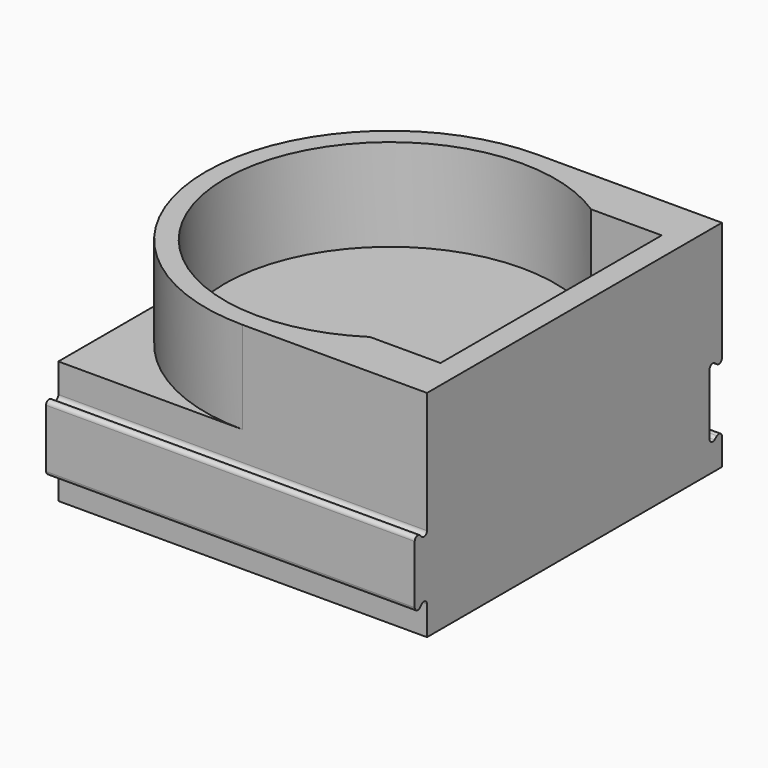
from build123d import *

# Parameters (mm, degrees)
F1_DEPTH  = 16
F2_DEPTH  = 12
F3_W      = 44
F3_H      = 44
F4_DEPTH  = 2
F5_R      = 1.65
F6_DEPTH  = 25
F8_DEPTH  = 48
F9_DEPTH  = 48
F10_R     = 0.5
F11_W     = 1.8
F11_H     = 2.1
F14_DEPTH = 10


# Not quite as in the source:
# - a feature names something its author has since deleted; it is built from what else it names


with BuildPart() as f1:
    # F0 (on Top) → F1 (new body)
    with BuildSketch(Plane.XY):
        with BuildLine():
            ThreePointArc((0, 24), (8.4852813742, 22.4499443206), (15.8745078664, 18))
            Line((15.8745078664, 18), (20.9579760163, 18))
            Line((20.9579760163, 18), (20.9579760163, 11.6945817069))
            ThreePointArc((20.9579760163, 11.6945817069), (23.2270469969, 6.0418778376), (24, 0))
            Line((24, 0), (24, 24))
            Line((24, 24), (0, 24))
        make_face()
        with BuildLine():
            Line((20.9579760163, -18), (15.8745078664, -18))
            ThreePointArc((15.8745078664, -18), (8.4852813742, -22.4499443206), (0, -24))
            Line((0, -24), (24, -24))
            Line((24, -24), (24, 0))
            ThreePointArc((24, 0), (23.2270469969, -6.0418778376), (20.9579760163, -11.6945817069))
            Line((20.9579760163, -11.6945817069), (20.9579760163, -18))
        make_face()
        with BuildLine():
            Line((15.8745078664, 18), (11.7579760163, 18))
            ThreePointArc((11.7579760163, 18), (17.6397784352, 12.2917946922), (20.9579760163, 4.7972118256))
            Line((20.9579760163, 4.7972118256), (20.9579760163, 11.6945817069))
            ThreePointArc((20.9579760163, 11.6945817069), (18.6841521671, 15.0632817737), (15.8745078664, 18))
        make_face()
        with BuildLine():
            ThreePointArc((11.7579760163, -18), (-21.5, 0), (11.7579760163, 18))
            Line((11.7579760163, 18), (15.8745078664, 18))
            ThreePointArc((15.8745078664, 18), (8.4852813742, 22.4499443206), (0, 24))
            ThreePointArc((0, 24), (-16.9705627485, 16.9705627485), (-24, 0))
            ThreePointArc((-24, 0), (-16.9705627485, -16.9705627485), (0, -24))
            ThreePointArc((0, -24), (8.4852813742, -22.4499443206), (15.8745078664, -18))
            Line((15.8745078664, -18), (11.7579760163, -18))
        make_face()
        with BuildLine():
            ThreePointArc((20.9579760163, -4.7972118256), (17.6397784352, -12.2917946922), (11.7579760163, -18))
            Line((11.7579760163, -18), (15.8745078664, -18))
            ThreePointArc((15.8745078664, -18), (18.6841521671, -15.0632817737), (20.9579760163, -11.6945817069))
            Line((20.9579760163, -11.6945817069), (20.9579760163, -4.7972118256))
        make_face()
        with BuildLine():
            Line((20.9579760163, 11.6945817069), (20.9579760163, 4.7972118256))
            ThreePointArc((20.9579760163, 4.7972118256), (21.364064271, 2.4138678143), (21.5, 0))
            ThreePointArc((21.5, 0), (21.364064271, -2.4138678143), (20.9579760163, -4.7972118256))
            Line((20.9579760163, -4.7972118256), (20.9579760163, -11.6945817069))
            ThreePointArc((20.9579760163, -11.6945817069), (23.2270469969, -6.0418778376), (24, 0))
            ThreePointArc((24, 0), (23.2270469969, 6.0418778376), (20.9579760163, 11.6945817069))
        make_face()
        with BuildLine():
            ThreePointArc((-24, 0), (-16.9705627485, 16.9705627485), (0, 24))
            Line((0, 24), (-24, 24))
            Line((-24, 24), (-24, 0))
        make_face()
        with BuildLine():
            Line((11.7579760163, -18), (11.7579760163, 18))
            ThreePointArc((11.7579760163, 18), (-21.5, 0), (11.7579760163, -18))
        make_face()
        with BuildLine():
            Line((-24, -24), (0, -24))
            ThreePointArc((0, -24), (-16.9705627485, -16.9705627485), (-24, 0))
            Line((-24, 0), (-24, -24))
        make_face()
        with BuildLine():
            Line((20.9579760163, 18), (15.8745078664, 18))
            ThreePointArc((15.8745078664, 18), (18.6841521671, 15.0632817737), (20.9579760163, 11.6945817069))
            Line((20.9579760163, 11.6945817069), (20.9579760163, 18))
        make_face()
        with BuildLine():
            ThreePointArc((20.9579760163, -11.6945817069), (18.6841521671, -15.0632817737), (15.8745078664, -18))
            Line((15.8745078664, -18), (20.9579760163, -18))
            Line((20.9579760163, -18), (20.9579760163, -11.6945817069))
        make_face()
        with BuildLine():
            ThreePointArc((21.5, 0), (21.364064271, 2.4138678143), (20.9579760163, 4.7972118256))
            Line((20.9579760163, 4.7972118256), (20.9579760163, -4.7972118256))
            ThreePointArc((20.9579760163, -4.7972118256), (21.364064271, -2.4138678143), (21.5, 0))
        make_face()
        with BuildLine():
            ThreePointArc((20.9579760163, 4.7972118256), (17.6397784352, 12.2917946922), (11.7579760163, 18))
            Line((11.7579760163, 18), (11.7579760163, -18))
            ThreePointArc((11.7579760163, -18), (17.6397784352, -12.2917946922), (20.9579760163, -4.7972118256))
            Line((20.9579760163, -4.7972118256), (20.9579760163, 4.7972118256))
        make_face()
    extrude(amount=-F1_DEPTH)

    # F0 (on Top) → F2 (join)
    with BuildSketch(Plane.XY):
        with BuildLine():
            ThreePointArc((11.7579760163, -18), (-21.5, 0), (11.7579760163, 18))
            Line((11.7579760163, 18), (15.8745078664, 18))
            ThreePointArc((15.8745078664, 18), (8.4852813742, 22.4499443206), (0, 24))
            ThreePointArc((0, 24), (-16.9705627485, 16.9705627485), (-24, 0))
            ThreePointArc((-24, 0), (-16.9705627485, -16.9705627485), (0, -24))
            ThreePointArc((0, -24), (8.4852813742, -22.4499443206), (15.8745078664, -18))
            Line((15.8745078664, -18), (11.7579760163, -18))
        make_face()
        with BuildLine():
            Line((20.9579760163, -18), (15.8745078664, -18))
            ThreePointArc((15.8745078664, -18), (8.4852813742, -22.4499443206), (0, -24))
            Line((0, -24), (24, -24))
            Line((24, -24), (24, 0))
            ThreePointArc((24, 0), (23.2270469969, -6.0418778376), (20.9579760163, -11.6945817069))
            Line((20.9579760163, -11.6945817069), (20.9579760163, -18))
        make_face()
        with BuildLine():
            Line((20.9579760163, 11.6945817069), (20.9579760163, 4.7972118256))
            ThreePointArc((20.9579760163, 4.7972118256), (21.364064271, 2.4138678143), (21.5, 0))
            ThreePointArc((21.5, 0), (21.364064271, -2.4138678143), (20.9579760163, -4.7972118256))
            Line((20.9579760163, -4.7972118256), (20.9579760163, -11.6945817069))
            ThreePointArc((20.9579760163, -11.6945817069), (23.2270469969, -6.0418778376), (24, 0))
            ThreePointArc((24, 0), (23.2270469969, 6.0418778376), (20.9579760163, 11.6945817069))
        make_face()
        with BuildLine():
            ThreePointArc((0, 24), (8.4852813742, 22.4499443206), (15.8745078664, 18))
            Line((15.8745078664, 18), (20.9579760163, 18))
            Line((20.9579760163, 18), (20.9579760163, 11.6945817069))
            ThreePointArc((20.9579760163, 11.6945817069), (23.2270469969, 6.0418778376), (24, 0))
            Line((24, 0), (24, 24))
            Line((24, 24), (0, 24))
        make_face()
        with BuildLine():
            ThreePointArc((21.5, 0), (21.364064271, 2.4138678143), (20.9579760163, 4.7972118256))
            Line((20.9579760163, 4.7972118256), (20.9579760163, -4.7972118256))
            ThreePointArc((20.9579760163, -4.7972118256), (21.364064271, -2.4138678143), (21.5, 0))
        make_face()
    extrude(amount=F2_DEPTH)

    # F3 (on face) → F4 (cut)
    with BuildSketch(Plane(origin=(0, 0, -16), x_dir=(1, 0, 0), z_dir=(0, 0, -1))):
        Rectangle(F3_W, F3_H)
    extrude(amount=-F4_DEPTH, mode=Mode.SUBTRACT)

    # F5 (on face) → F6 (cut)
    with BuildSketch(Plane(origin=(0, 0, -14), x_dir=(1, 0, 0), z_dir=(0, 0, -1))):
        with BuildLine():
            ThreePointArc((17.3732751343, 12.6656745224), (16.7780906851, 13.4441687345), (16.1480507184, 14.1947334599))
            ThreePointArc((16.1480507184, 14.1947334599), (14.4166793265, 11.5940731357), (17.3745826654, 12.6))
            ThreePointArc((17.3745826654, 12.6), (17.3742557502, 12.6328437686), (17.3732751343, 12.6656745224))
        make_face()
        with BuildLine():
            ThreePointArc((17.3732751343, 12.6656745224), (17.0122035784, 13.6317617866), (16.1480507184, 14.1947334599))
            ThreePointArc((16.1480507184, 14.1947334599), (16.7780906851, 13.4441687345), (17.3732751343, 12.6656745224))
        make_face()
        with Locations((15.7245826654, 6.3)):
            Circle(F5_R)
        with Locations((15.7245826654, 0)):
            Circle(F5_R)
        with Locations((15.7245826654, -6.3)):
            Circle(F5_R)
        with BuildLine():
            ThreePointArc((17.3732751343, -12.6656745224), (16.7780906851, -13.4441687345), (16.1480507184, -14.1947334599))
            ThreePointArc((16.1480507184, -14.1947334599), (17.0122035784, -13.6317617866), (17.3732751343, -12.6656745224))
        make_face()
        with BuildLine():
            ThreePointArc((17.3745826654, -12.6), (14.4166793265, -11.5940731357), (16.1480507184, -14.1947334599))
            ThreePointArc((16.1480507184, -14.1947334599), (16.7780906851, -13.4441687345), (17.3732751343, -12.6656745224))
            ThreePointArc((17.3732751343, -12.6656745224), (17.3742557502, -12.6328437686), (17.3745826654, -12.6))
        make_face()
    extrude(amount=-F6_DEPTH, mode=Mode.SUBTRACT)

    # F7 (on face) → F8 (join, through all)
    with BuildSketch(Plane.YZ.offset(24)):
        Polygon((-26, -13), (-24, -11), (-24, -5), (-26, -3), align=None)
    extrude(amount=-F8_DEPTH)

    # F7 (on face) → F9 (cut, through all)
    with BuildSketch(Plane.YZ.offset(24)):
        Polygon((22, -13), (24, -11.4928918998), (24, -4.5071081002), (22, -3), align=None)
    extrude(amount=-F9_DEPTH, mode=Mode.SUBTRACT)

    # F10
    f10_edges = [f1.edges().sort_by_distance(p)[0] for p in [
        (0, -26, -13),
        (0, -26, -3),
        (0, 22, -3),
        (0, 22, -13),
        (0, 24, -4.507108),
        (0, 24, -11.492892),
        (0, -24, -5),
        (0, -24, -11),
    ]]
    fillet(f10_edges, radius=F10_R)

    # F11 (on Front) → F12 (revolve, cut)
    with BuildSketch(Plane.XZ):
        with Locations((12.6579760163, 5.05)):
            Rectangle(F11_W, F11_H)
    revolve(axis=Axis((0, 0, 12), (0, 0, -1)), mode=Mode.SUBTRACT)

    # F0 (on Top) + F13 (on face) → F14 (cut)
    with BuildSketch(Plane.XY):
        with BuildLine():
            ThreePointArc((20.9579760163, 4.7972118256), (17.6397784352, 12.2917946922), (11.7579760163, 18))
            Line((11.7579760163, 18), (11.7579760163, -18))
            ThreePointArc((11.7579760163, -18), (17.6397784352, -12.2917946922), (20.9579760163, -4.7972118256))
            Line((20.9579760163, -4.7972118256), (20.9579760163, 4.7972118256))
        make_face()
        with BuildLine():
            ThreePointArc((20.9579760163, -4.7972118256), (17.6397784352, -12.2917946922), (11.7579760163, -18))
            Line((11.7579760163, -18), (15.8745078664, -18))
            ThreePointArc((15.8745078664, -18), (18.6841521671, -15.0632817737), (20.9579760163, -11.6945817069))
            Line((20.9579760163, -11.6945817069), (20.9579760163, -4.7972118256))
        make_face()
        with BuildLine():
            ThreePointArc((20.9579760163, -11.6945817069), (18.6841521671, -15.0632817737), (15.8745078664, -18))
            Line((15.8745078664, -18), (20.9579760163, -18))
            Line((20.9579760163, -18), (20.9579760163, -11.6945817069))
        make_face()
    with BuildSketch(Plane.XY):
        with BuildLine():
            Line((20.9579760163, 18), (11.7579760163, 18))
            ThreePointArc((11.7579760163, 18), (17.6397784352, 12.2917946922), (20.9579760163, 4.7972118256))
            Line((20.9579760163, 4.7972118256), (20.9579760163, 18))
        make_face()
    extrude(amount=-F14_DEPTH, mode=Mode.SUBTRACT)


solid = f1.part
